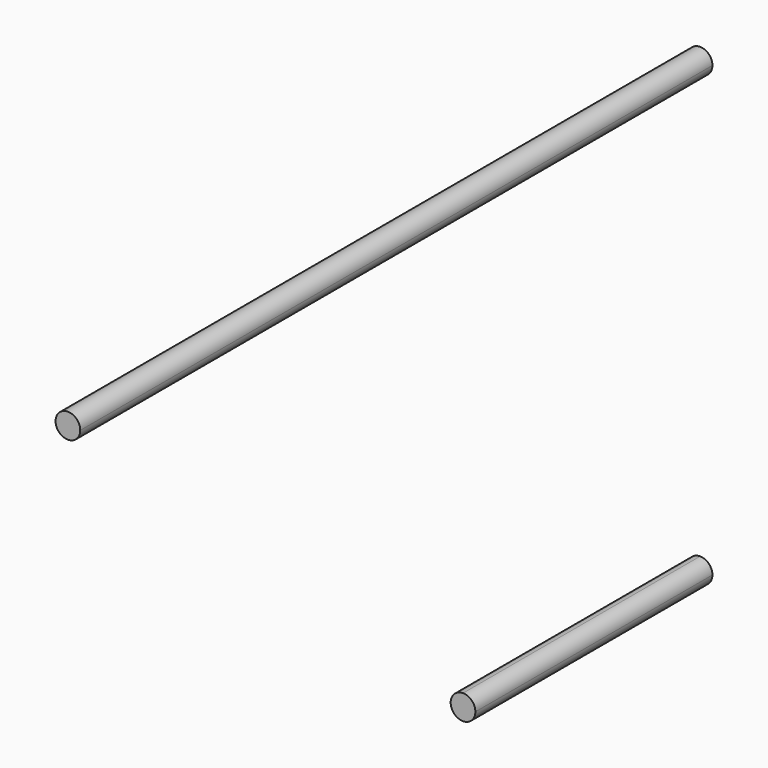
from build123d import *

# Parameters (mm, degrees)
F1_DEPTH = 101.6
F2_DEPTH = 38.1


# Not quite as in the source:
# - the program builds the solid bodies; features that only make, move or delete a surface that nothing else refers to are left out


with BuildPart() as f1:
    # F0 (on Front) → F1 (new body)
    with BuildSketch(Plane.XZ):
        with BuildLine():
            ThreePointArc((1.5875, 8.5184694223), (-1.1225320151, 9.6410014374), (0, 6.9309694223))
            ThreePointArc((0, 6.9309694223), (1.1225320151, 7.3959374071), (1.5875, 8.5184694223))
        make_face()
    extrude(amount=F1_DEPTH)


with BuildPart() as f2:
    # F0 (on Front) → F2 (new body)
    with BuildSketch(Plane.XZ):
        with BuildLine():
            ThreePointArc((1.5875, -49.1515211761), (1.1225320151, -48.028989161), (0, -47.5640211761))
            ThreePointArc((0, -47.5640211761), (-1.1225320151, -50.2740531912), (1.5875, -49.1515211761))
        make_face()
    extrude(amount=F2_DEPTH)


solid = Compound([f1.part, f2.part])
